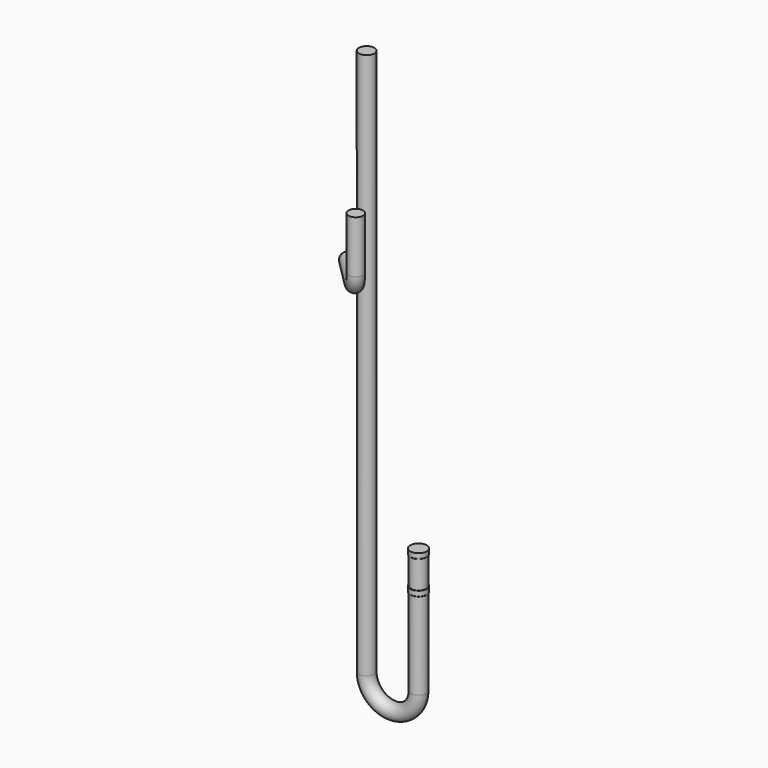
from build123d import *

# Parameters (mm, degrees)
F4_SIZE   = 0.99999
F6_R      = 14
F7_DEPTH  = 990
F3_FACE_R = 14
F11_R     = 13.0604129179


# Not quite as in the source:
# - a fillet or chamfer is up to 0.001 mm smaller than in the source, because OpenCascade refuses the exact size


with BuildPart() as f3:
    # F2 (on Front) → F3 (revolve)
    with BuildSketch(Plane.XZ):
        Polygon((0, 302), (0, 75), (14, 75), (14, 232), (15, 232), (15, 242), (14, 242), (14, 292), (15, 292), (15, 302), align=None)
    revolve(axis=Axis((0, 0, 188.5), (0, 0, 1)))

    # F4 (size 1 in the source; OpenCascade refuses exactly that, so slightly less here)
    f4_edges = [f3.edges().sort_by_distance(p)[0] for p in [
        (-15, 0, 232),
        (-15, 0, 292),
    ]]
    chamfer(f4_edges, length=F4_SIZE)



with BuildPart() as f7:
    # F6 (on face) → F7 (new body)
    with BuildSketch(Plane(origin=(0, 0, 75), x_dir=(1, 0, 0), z_dir=(0, 0, -1))):
        with Locations((-94, 0)):
            Circle(F6_R)
    extrude(amount=-F7_DEPTH)


with BuildPart() as f3_1:
    add(f3.part)

    add(f7.part)  # F9 merges F7
    # F9: sweep along a path in F8
    with BuildLine(Plane.XZ) as f9_path:
        ThreePointArc((-94, 75), (-47, 28), (0, 75))
    # F3_face (on face) → F9 (sweep)
    with BuildSketch(Plane(origin=(0, 0, 75), x_dir=(1, 0, 0), z_dir=(0, 0, -1))):
        Circle(F3_FACE_R)
    sweep(path=f9_path.line)


with BuildPart() as f14:
    # F14: sweep along a path in F13
    with BuildLine(Plane(origin=(-69.5, -69.5, 0), x_dir=(-0.7071067812, 0.7071067812, 0), z_dir=(0.7071067812, 0.7071067812, 0))) as f14_path:
        Line((-80.7121574151, 884), (-80.7121574151, 789))
        ThreePointArc((-80.7121574151, 789), (-71.9253608507, 767.7867965644), (-50.7121574151, 759))
        Line((-50.7121574151, 759), (18.2878425849, 759))
    # F11 (on offset) → F14 (sweep)
    with BuildSketch(Plane.XY.offset(884)):
        with Locations((-12.4278861676, -126.5721138324)):
            Circle(F11_R)
    sweep(path=f14_path.line)


solid = Compound([f3_1.part, f14.part])
